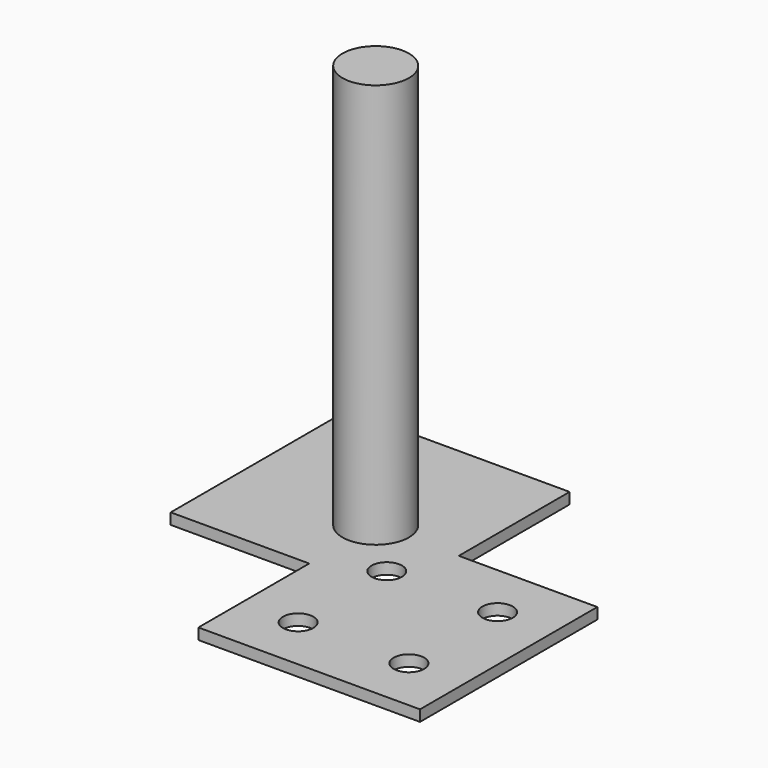
from build123d import *

# Parameters (mm, degrees)
F0_R     = 5.5
F0_R_2   = 12
F1_DEPTH = 4
F2_R     = 12
F3_DEPTH = 150


with BuildPart() as f1:
    # F0 (on Top) → F1 (new body)
    with BuildSketch(Plane.XY):
        Polygon((30, 50), (-50, 50), (-50, -30), (0, -30), (0, -80), (80, -80), (80, 0), (30, 0), align=None)
        with Locations((20, -60)):
            Circle(F0_R, mode=Mode.SUBTRACT)
        with Locations((60, -60)):
            Circle(F0_R, mode=Mode.SUBTRACT)
        with Locations((20, -20)):
            Circle(F0_R, mode=Mode.SUBTRACT)
        with Locations((60, -20)):
            Circle(F0_R, mode=Mode.SUBTRACT)
        Circle(F0_R_2, mode=Mode.SUBTRACT)
    extrude(amount=F1_DEPTH)

    # F2 (on face) → F3 (join)
    with BuildSketch(Plane(origin=(0, 0, 0), x_dir=(1, 0, 0), z_dir=(0, 0, -1))):
        Circle(F2_R)
    extrude(amount=-F3_DEPTH)


solid = f1.part
